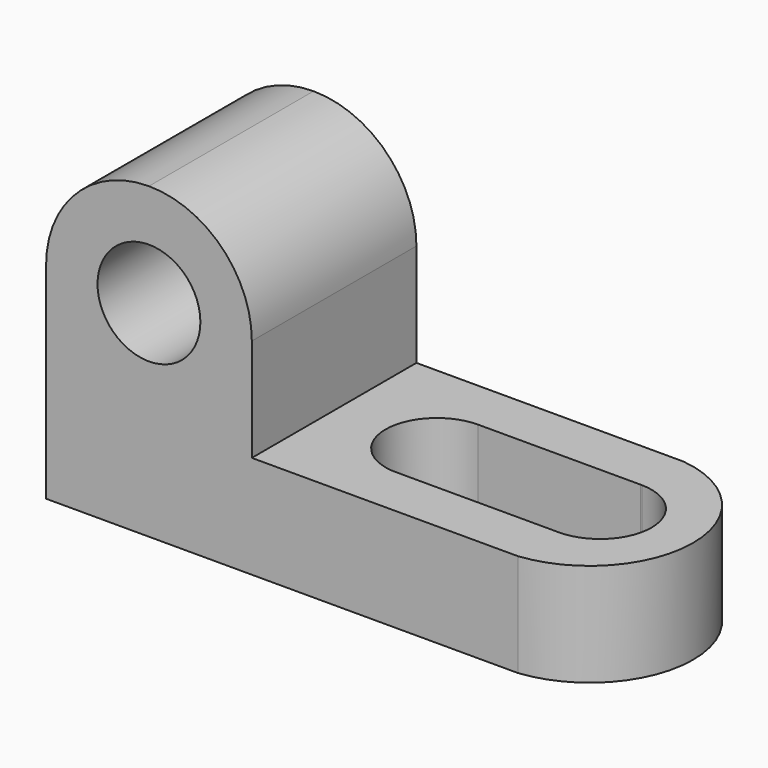
from build123d import *

# Parameters (mm, degrees)
F1_DEPTH = 25.4
F2_R     = 6.35
F3_DEPTH = 25.401
F5_DEPTH = 25.401
F7_DEPTH = 12.701


# Not quite as in the source:
# - a feature names something its author has since deleted; it is built from what else it names


with BuildPart() as f1:
    # F0 (on Front) → F1 (new body)
    with BuildSketch(Plane.XZ):
        Polygon((-46.455263897, 38.1), (-71.855263897, 38.1), (-71.855263897, 0), (-2.005263897, 0), (-2.005263897, 12.7), (-46.455263897, 12.7), align=None)
    extrude(amount=F1_DEPTH)

    # F2 (on face) → F3 (cut, through all)
    with BuildSketch(Plane.XZ.offset(25.4)):
        with Locations((-59.155263897, 25.4)):
            Circle(F2_R)
    extrude(amount=-F3_DEPTH, mode=Mode.SUBTRACT)

    # F4 (on face) → F5 (cut, through all)
    with BuildSketch(Plane.XZ.offset(25.4)):
        with BuildLine():
            ThreePointArc((-71.855263897, 25.4), (-68.135520018, 34.3802561211), (-59.155263897, 38.1))
            Line((-59.155263897, 38.1), (-71.855263897, 38.1))
            Line((-71.855263897, 38.1), (-71.855263897, 25.4))
        make_face()
        with BuildLine():
            ThreePointArc((-59.155263897, 38.1), (-50.1750077759, 34.3802561211), (-46.455263897, 25.4))
            Line((-46.455263897, 25.4), (-46.455263897, 38.1))
            Line((-46.455263897, 38.1), (-59.155263897, 38.1))
        make_face()
    extrude(amount=-F5_DEPTH, mode=Mode.SUBTRACT)

    # F6 (on face) → F7 (cut, through all)
    with BuildSketch(Plane.XY.offset(12.7)):
        with BuildLine():
            ThreePointArc((-13.507871342, -6.3510340362), (-13.6221384518, -6.3500000083), (-13.7364056666, -6.3510223648))
            Line((-13.7364056666, -6.3510223648), (-13.507871342, -6.3510340362))
        make_face()
        with BuildLine():
            Line((-13.507871342, -6.3510340362), (-13.7364056666, -6.3510223648))
            ThreePointArc((-13.7364056666, -6.3510223648), (-19.9722112621, -12.7565139443), (-13.6233824013, -19.0499999334))
            ThreePointArc((-13.6233824013, -19.0499999334), (-9.1326598467, -17.1904531948), (-7.2724627495, -12.7))
            ThreePointArc((-7.2724627495, -12.7), (-9.0920016561, -8.2505705668), (-13.507871342, -6.3510340362))
        make_face()
        with BuildLine():
            ThreePointArc((-33.7549395993, -6.3500000083), (-29.2650211814, -8.2099865975), (-27.405263897, -12.7))
            ThreePointArc((-27.405263897, -12.7), (-29.1979362777, -17.1219073906), (-33.5637725492, -19.0471120255))
            Line((-33.5637725492, -19.0471120255), (-13.6233824013, -19.0499999334))
            ThreePointArc((-13.6233824013, -19.0499999334), (-19.9722112621, -12.7565139443), (-13.7364056666, -6.3510223648))
            Line((-13.7364056666, -6.3510223648), (-33.7549395993, -6.3500000083))
        make_face()
        with BuildLine():
            ThreePointArc((-33.5637725492, -19.0471120255), (-29.1979362777, -17.1219073906), (-27.405263897, -12.7))
            ThreePointArc((-27.405263897, -12.7), (-29.2650211814, -8.2099865975), (-33.7549395993, -6.3500000083))
            ThreePointArc((-33.7549395993, -6.3500000083), (-40.1045443054, -12.7955944315), (-33.5637725492, -19.0471120255))
        make_face()
        with BuildLine():
            ThreePointArc((-13.507871342, 0), (-2.1464755419, -12.7515151154), (-13.6224627495, -25.4))
            Line((-13.6224627495, -25.4), (-2.005263897, -25.4))
            Line((-2.005263897, -25.4), (-2.005263897, 0))
            Line((-2.005263897, 0), (-13.507871342, 0))
        make_face()
    extrude(amount=-F7_DEPTH, mode=Mode.SUBTRACT)


solid = f1.part
